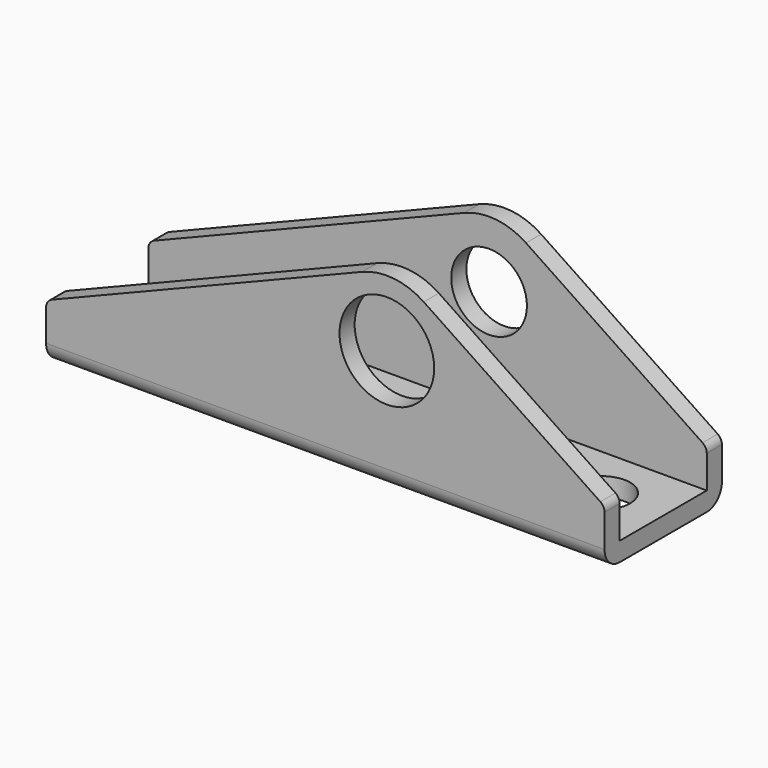
from build123d import *

# Parameters (mm, degrees)
F0_R     = 5
F0_R_2   = 4
F1_DEPTH = 15.5
F2_W     = 11.5
F2_H     = 26.2481089791
F2_H_2   = 4
F3_DEPTH = 59.001
F4_R     = 3
F5_DEPTH = 2
F6_R     = 1
F7_R     = 2
F8_R     = 5
F8_R_2   = 4
F9_DEPTH = 2


# Not quite as in the source:
# - a feature names something its author has since deleted; it is built from what else it names


with BuildPart() as f1:
    # F0 (on Front) → F1 (new body)
    with BuildSketch(Plane.XZ):
        with BuildLine():
            Line((-36, -7), (-4.54e-08, -7))
            ThreePointArc((-4.54e-08, -7), (-6.871307732, -1.3360875914), (-2.6230483271, 6.4899628253))
            Line((-2.6230483271, 6.4899628253), (-36, -7))
        make_face()
        Polygon((23, -7), (-4.54e-08, -7), (-36, -7), (-36, -13), (23, -13), align=None)
        with BuildLine():
            ThreePointArc((3.8996539792, 5.8131487889), (6.1764705882, 3.2941176471), (7, 0))
            ThreePointArc((7, 0), (4.9497474522, -4.9497474844), (-4.54e-08, -7))
            Line((-4.54e-08, -7), (23, -7))
            Line((23, -7), (3.8996539792, 5.8131487889))
        make_face()
        with BuildLine():
            ThreePointArc((-4.54e-08, -7), (4.9497474522, -4.9497474844), (7, 0))
            ThreePointArc((7, 0), (6.1764705882, 3.2941176471), (3.8996539792, 5.8131487889))
            ThreePointArc((3.8996539792, 5.8131487889), (0.7224609385, 6.9626180559), (-2.6230483271, 6.4899628253))
            ThreePointArc((-2.6230483271, 6.4899628253), (-6.871307732, -1.3360875914), (-4.54e-08, -7))
        make_face()
        Circle(F0_R, mode=Mode.SUBTRACT)
        Circle(F0_R)
        Circle(F0_R_2, mode=Mode.SUBTRACT)
    extrude(amount=F1_DEPTH)

    # F2 (on face) → F3 (cut, through all)
    with BuildSketch(Plane.YZ.offset(23)):
        with Locations((-7.75, 6.1240544895)):
            Rectangle(F2_W, F2_H)
        with Locations((-7.75, -9)):
            Rectangle(F2_W, F2_H_2)
    extrude(amount=-F3_DEPTH, mode=Mode.SUBTRACT)

    # F4 (on face) → F5 (cut)
    with BuildSketch(Plane(origin=(0, 0, -13), x_dir=(1, 0, 0), z_dir=(0, 0, -1))):
        with BuildLine():
            ThreePointArc((-29, 4.75), (-26.8786796564, 5.6286796564), (-26, 7.75))
            ThreePointArc((-26, 7.75), (-26.8786796564, 9.8713203436), (-29, 10.75))
            ThreePointArc((-29, 10.75), (-32, 7.75), (-29, 4.75))
        make_face()
        with BuildLine():
            ThreePointArc((-29, 10.75), (-26.8786796564, 9.8713203436), (-26, 7.75))
            ThreePointArc((-26, 7.75), (-26.8786796564, 5.6286796564), (-29, 4.75))
            Line((-29, 4.75), (-20.5, 4.75))
            ThreePointArc((-20.5, 4.75), (-23.5, 7.75), (-20.5, 10.75))
            Line((-20.5, 10.75), (-29, 10.75))
        make_face()
        with BuildLine():
            ThreePointArc((-17.5, 7.75), (-18.3786796564, 9.8713203436), (-20.5, 10.75))
            ThreePointArc((-20.5, 10.75), (-23.5, 7.75), (-20.5, 4.75))
            ThreePointArc((-20.5, 4.75), (-18.3786796564, 5.6286796564), (-17.5, 7.75))
        make_face()
        with Locations((16.5, 7.75)):
            Circle(F4_R)
    extrude(amount=-F5_DEPTH, mode=Mode.SUBTRACT)

    # F6
    f6_edges = [f1.edges().sort_by_distance(p)[0] for p in [
        (-36, -14.5, -7),
        (-36, -1, -7),
        (23, -14.5, -7),
        (23, -1, -7),
    ]]
    fillet(f6_edges, radius=F6_R)

    # F7
    f7_edges = [f1.edges().sort_by_distance(p)[0] for p in [
        (-6.5, -15.5, -13),
        (-6.5, 0, -13),
    ]]
    fillet(f7_edges, radius=F7_R)

    # F8 (on face) → F9 (cut, through all)
    with BuildSketch(Plane.XZ.offset(15.5)):
        Circle(F8_R)
        Circle(F8_R_2, mode=Mode.SUBTRACT)
    extrude(amount=-F9_DEPTH, mode=Mode.SUBTRACT)


solid = f1.part
